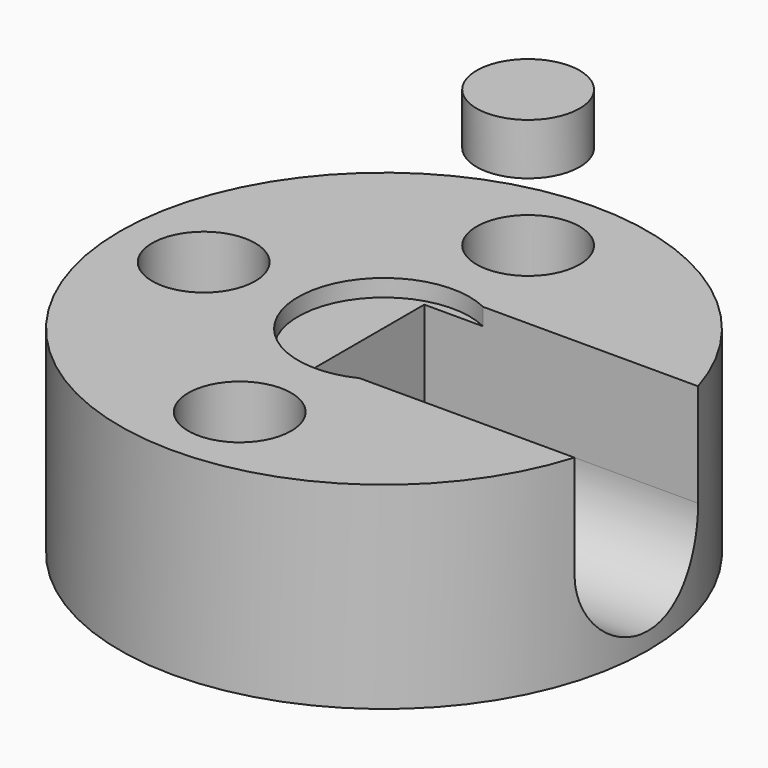
from build123d import *

# Parameters (mm, degrees)
F0_R          = 30.75
F1_DEPTH      = 23
F4_DEPTH      = 31.7500001
F4_DEPTH_BACK = 2.5
F5_R          = 6
F6_DEPTH      = 22
F7_DEPTH      = 22
F9_D          = 5
F9_DEPTH      = 9.5
F9_TIP        = 1.5021515476
F10_R         = 10
F11_DEPTH     = 2
F13_R         = 6
F14_DEPTH     = 6


# Not quite as in the source:
# - a pattern or mirror of a feature is missing from the dataset's text; its kind, count and spacing are read off the source's solid


with BuildPart() as f1:
    # F0 (on Top) → F1 (new body)
    with BuildSketch(Plane.XY):
        Circle(F0_R)
    extrude(amount=F1_DEPTH)

    # F3 (on Right) → F4 (cut, two sides)
    with BuildSketch(Plane.YZ) as f4_sk:
        with BuildLine():
            Line((9, 11), (9, 44))
            Line((9, 44), (-9, 44))
            Line((-9, 44), (-9, 11))
            ThreePointArc((-9, 11), (-6.3639610307, 4.6360389693), (0, 2))
            ThreePointArc((0, 2), (6.3639610307, 4.6360389693), (9, 11))
        make_face()
    extrude(amount=F4_DEPTH, mode=Mode.SUBTRACT)
    extrude(f4_sk.sketch, amount=-F4_DEPTH_BACK, mode=Mode.SUBTRACT)

    # F5 (on face) → F6 (cut)
    with BuildSketch(Plane.XY.offset(23)):
        with Locations((0, 21)):
            Circle(F5_R)
    f6 = extrude(amount=-F6_DEPTH, mode=Mode.SUBTRACT)

    # F6_copies: F6 across plane
    add(f6.mirror(Plane(origin=(0, 0, 0), x_dir=(0, 0, -1), z_dir=(0, -1, 0))), mode=Mode.SUBTRACT)

    # F5 (on face) → F7 (cut)
    with BuildSketch(Plane.XY.offset(23)):
        with Locations((-21, 0)):
            Circle(F5_R)
    extrude(amount=-F7_DEPTH, mode=Mode.SUBTRACT)

    # F9
    with Locations(Plane.YZ.offset(-2.5)):
        with Locations((0, 11)):
            Hole(F9_D / 2, depth=F9_DEPTH)
            with Locations((0, 0, -(F9_DEPTH + F9_TIP / 2))):  # 118° drill point
                Cone(0, F9_D / 2, F9_TIP, mode=Mode.SUBTRACT)

    # F10 (on face) → F11 (cut)
    with BuildSketch(Plane.XY.offset(23)):
        Circle(F10_R)
    extrude(amount=-F11_DEPTH, mode=Mode.SUBTRACT)


with BuildPart() as f14:
    # F13 (on offset) → F14 (new body)
    with BuildSketch(Plane.XY.offset(33)):
        with Locations((0, 21)):
            Circle(F13_R)
    extrude(amount=F14_DEPTH)


solid = Compound([f1.part, f14.part])
